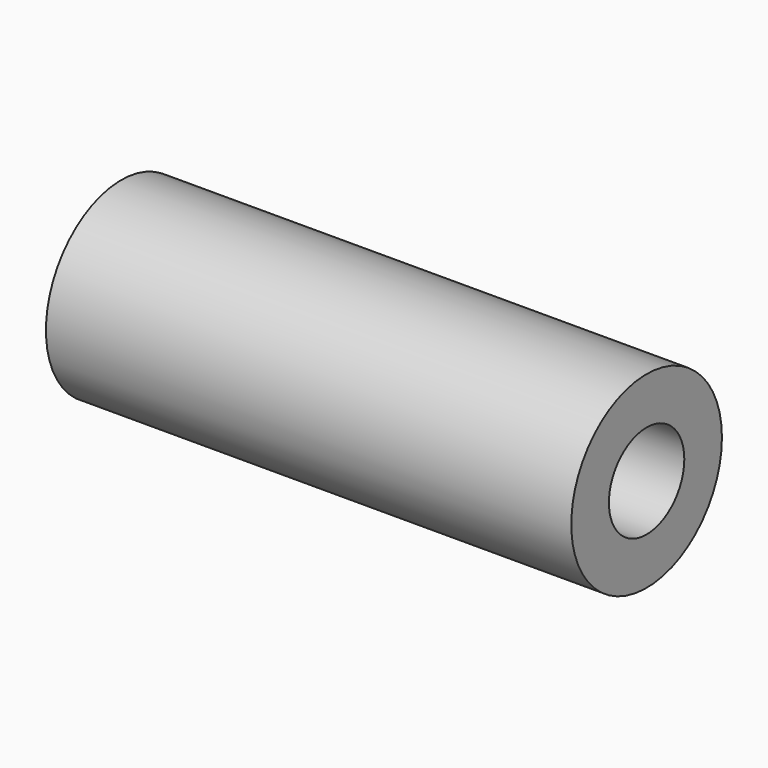
from build123d import *

# Parameters (mm, degrees)
F0_R     = 7.3291649142
F1_DEPTH = 40.894
F2_R     = 3.66881969
F3_DEPTH = 81.534


# Not quite as in the source:
# - a feature names something its author has since deleted; it is built from what else it names


with BuildPart() as f1:
    # F0 (on Right) → F1 (new body)
    with BuildSketch(Plane.YZ):
        Circle(F0_R)
    extrude(amount=-F1_DEPTH)

    # F2 (on Right) → F3 (cut)
    with BuildSketch(Plane.YZ):
        Circle(F2_R)
    extrude(amount=-F3_DEPTH, mode=Mode.SUBTRACT)


solid = f1.part
